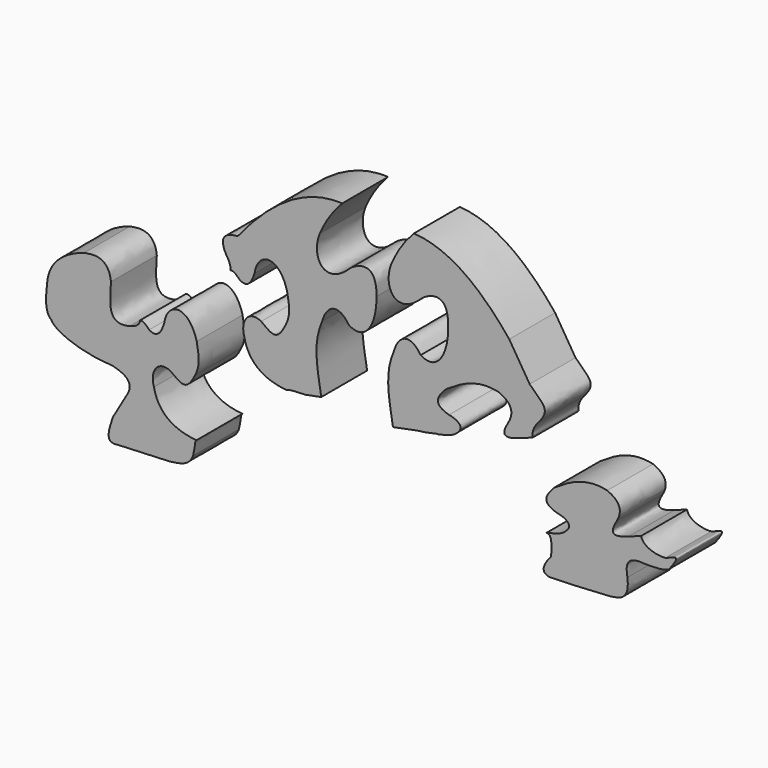
from build123d import *

# Parameters (mm, degrees)
F1_DEPTH = 12


with BuildPart() as f1:
    # F0 (on Front) → F1 (new body)
    with BuildSketch(Plane.XZ):
        with BuildLine():
            add(Edge.make_bspline(
                [(-45.8449507755, -30.2722072455), (-45.0373038776, -30.1761162576), (-44.6484686549, -30.7578016467), (-43.941360189, -31.4056891493)],
                knots=[0.0138164207, 0.0138164207, 0.0138164207, 0.0138164207, 0.9928004802, 0.9928004802, 0.9928004802, 0.9928004802], degree=3))
            add(Edge.make_bspline(
                [(-48.0757471404, -32.0822951013), (-46.6881017023, -31.7283579413), (-45.9495435845, -31.1383058377), (-45.8449507755, -30.2722072455)],
                knots=[0, 0, 0, 0, 0.5631001463, 0.5631001463, 0.5631001463, 0.5631001463], degree=3))
            add(Edge.make_bspline(
                [(-51.9596131404, -25.1498021013), (-52.0998001404, -29.0032331013), (-52.9532851404, -33.2183801013), (-48.0757471404, -32.0822951013)],
                knots=[0, 0, 0, 0, 1, 1, 1, 1], degree=3))
            add(Edge.make_bspline(
                [(-57.5557201404, -21.6417971013), (-56.1260271404, -21.4227111013), (-52.4818251404, -20.5015511013), (-51.9596131404, -25.1498021013)],
                knots=[0, 0, 0, 0, 1, 1, 1, 1], degree=3))
            add(Edge.make_bspline(
                [(-65.3234511404, -29.8271471013), (-65.0594941404, -25.9076961013), (-62.3853321404, -23.2227411013), (-57.5557201404, -21.6417971013)],
                knots=[0, 0, 0, 0, 1, 1, 1, 1], degree=3))
            add(Edge.make_bspline(
                [(-64.4464501404, -36.2167321013), (-65.7482111404, -35.2981831013), (-65.6745951404, -32.7291821013), (-65.3234511404, -29.8271471013)],
                knots=[0, 0, 0, 0, 1, 1, 1, 1], degree=3))
            add(Edge.make_bspline(
                [(-51.5002301404, -40.5599791013), (-58.8537851404, -40.1618431013), (-63.7433521404, -37.8487831013), (-64.4464501404, -36.2167321013)],
                knots=[0, 0, 0, 0, 1, 1, 1, 1], degree=3))
            add(Edge.make_bspline(
                [(-48.3680811404, -44.4856091013), (-46.9755981404, -41.7222641013), (-50.1851831404, -40.9703021013), (-51.5002301404, -40.5599791013)],
                knots=[0, 0, 0, 0, 1, 1, 1, 1], degree=3))
            Line((-48.3680811404, -44.4856091013), (-51.5419931404, -49.9564301013))
            add(Edge.make_bspline(
                [(-50.6649911404, -54.7590591013), (-53.3456761404, -55.1932241013), (-52.4255291404, -52.5592301013), (-51.5419931404, -49.9564301013)],
                knots=[0, 0, 0, 0, 1, 1, 1, 1], degree=3))
            Line((-50.6649911404, -54.7590591013), (-39.6369361507, -54.2805532244))
            add(Edge.make_bspline(
                [(-34.7507801507, -51.6077842244), (-35.6369361507, -54.0036222244), (-37.8110571507, -53.9730942244), (-39.6369361507, -54.2805532244)],
                knots=[0, 0, 0, 0, 1, 1, 1, 1], degree=3))
            add(Edge.make_bspline(
                [(-34.0284567295, -48.5307527398), (-34.4745798989, -48.8886475977), (-34.2730056498, -49.6825430518), (-34.7507801507, -51.6077842244)],
                knots=[0.4766943603, 0.4766943603, 0.4766943603, 0.4766943603, 0.9954393419, 0.9954393419, 0.9954393419, 0.9954393419], degree=3))
            add(Edge.make_bspline(
                [(-42.959955189, -41.6373791493), (-42.0418390729, -46.1886284081), (-38.5284702823, -48.1795127961), (-34.0284567295, -48.5307527398)],
                knots=[0, 0, 0, 0, 0.9845136883, 0.9845136883, 0.9845136883, 0.9845136883], degree=3))
            add(Edge.make_bspline(
                [(-39.431065189, -37.6073471493), (-42.009885189, -36.2487441493), (-43.877970189, -38.7036141493), (-42.959955189, -41.6373791493)],
                knots=[0, 0, 0, 0, 1, 1, 1, 1], degree=3))
            add(Edge.make_bspline(
                [(-34.294339189, -36.5632971493), (-36.196497189, -40.4302951493), (-37.241376189, -39.1889491493), (-39.431065189, -37.6073471493)],
                knots=[0, 0, 0, 0, 1, 1, 1, 1], degree=3))
            add(Edge.make_bspline(
                [(-34.002007189, -30.3198791493), (-33.615278189, -32.3526011493), (-33.151711189, -34.3776391493), (-34.294339189, -36.5632971493)],
                knots=[0, 0, 0, 0, 1, 1, 1, 1], degree=3))
            add(Edge.make_bspline(
                [(-40.809210189, -29.1505421493), (-40.138114189, -24.6796841493), (-35.639198189, -24.2694741493), (-34.002007189, -30.3198791493)],
                knots=[0, 0, 0, 0, 1, 1, 1, 1], degree=3))
            add(Edge.make_bspline(
                [(-43.941360189, -31.4056891493), (-42.081064189, -32.5779841493), (-41.316846189, -30.7279271493), (-40.809210189, -29.1505421493)],
                knots=[0, 0, 0, 0, 1, 1, 1, 1], degree=3))
        make_face()
    extrude(amount=F1_DEPTH)


with BuildPart() as f1b:
    # F0 (on Front) → F1, piece 2 (new body)
    with BuildSketch(Plane.XZ):
        with BuildLine():
            add(Edge.make_bspline(
                [(-3.5493105797, 5.0215643728), (-5.8036935797, 2.7199413728), (-7.1759255797, 0.3343053728), (-8.2684195797, -2.0779746272)],
                knots=[0, 0, 0, 0, 1, 1, 1, 1], degree=3))
            add(Edge.make_bspline(
                [(-25.4296236107, -8.1543007714), (-18.3372787343, 0.7478813145), (-11.0568971369, 5.4326630198), (-3.5493105797, 5.0215643728)],
                knots=[0, 0, 0, 0, 0.5368262438, 0.5368262438, 0.5368262438, 0.5368262438], degree=3))
            add(Edge.make_bspline(
                [(-27.8100566107, -12.3722607714), (-29.3184416107, -9.6427037714), (-28.3748066107, -8.3230577714), (-25.4296236107, -8.1543007714)],
                knots=[0, 0, 0, 0, 1, 1, 1, 1], degree=3))
            add(Edge.make_bspline(
                [(-26.9156442458, -14.9054209156), (-26.8344924591, -14.2334297064), (-27.134984297, -13.3952600313), (-27.8100566107, -12.3722607714)],
                knots=[0.5631001463, 0.5631001463, 0.5631001463, 0.5631001463, 1, 1, 1, 1], degree=3))
            add(Edge.make_bspline(
                [(-26.9156442458, -14.9054209156), (-26.1079973479, -14.8093299277), (-25.7191621253, -15.3910153168), (-25.0120536594, -16.0389028194)],
                knots=[0.0138164207, 0.0138164207, 0.0138164207, 0.0138164207, 0.9928004802, 0.9928004802, 0.9928004802, 0.9928004802], degree=3))
            add(Edge.make_bspline(
                [(-25.0120536594, -16.0389028194), (-23.1517576594, -17.2111978194), (-22.3875396594, -15.3611408194), (-21.8799036594, -13.7837558194)],
                knots=[0, 0, 0, 0, 1, 1, 1, 1], degree=3))
            add(Edge.make_bspline(
                [(-21.8799036594, -13.7837558194), (-21.2088076594, -9.3128978194), (-16.7098916594, -8.9026878194), (-15.0727006594, -14.9530928194)],
                knots=[0, 0, 0, 0, 1, 1, 1, 1], degree=3))
            add(Edge.make_bspline(
                [(-15.0727006594, -14.9530928194), (-14.6859716594, -16.9858148194), (-14.2224046594, -19.0108528194), (-15.3650326594, -21.1965108194)],
                knots=[0, 0, 0, 0, 1, 1, 1, 1], degree=3))
            add(Edge.make_bspline(
                [(-15.3650326594, -21.1965108194), (-17.2671906594, -25.0635088194), (-18.3120696594, -23.8221628194), (-20.5017586594, -22.2405608194)],
                knots=[0, 0, 0, 0, 1, 1, 1, 1], degree=3))
            add(Edge.make_bspline(
                [(-20.5017586594, -22.2405608194), (-23.0805786594, -20.8819578194), (-24.9486636594, -23.3368278194), (-24.0306486594, -26.2705928194)],
                knots=[0, 0, 0, 0, 1, 1, 1, 1], degree=3))
            add(Edge.make_bspline(
                [(-24.0306486594, -26.2705928194), (-23.1125325433, -30.8218420782), (-19.5991637527, -32.8127264662), (-15.0991501999, -33.1639664098)],
                knots=[0, 0, 0, 0, 0.9845136883, 0.9845136883, 0.9845136883, 0.9845136883], degree=3))
            add(Edge.make_bspline(
                [(-11.2265906851, -32.7437242637), (-13.7393281571, -32.8740949128), (-14.6907009874, -32.8362948542), (-15.0991501999, -33.1639664098)],
                knots=[0.0017560612, 0.0017560612, 0.0017560612, 0.0017560612, 0.4766943603, 0.4766943603, 0.4766943603, 0.4766943603], degree=3))
            Line((-11.2265906851, -32.7437242637), (-7.9269410512, -32.0941016145))
            add(Edge.make_bspline(
                [(-7.7255115797, -18.0310576272), (-9.8693992766, -22.8725708581), (-8.6456012061, -27.4646273112), (-7.9269410512, -32.0941016145)],
                knots=[0, 0, 0, 0, 0.9940362568, 0.9940362568, 0.9940362568, 0.9940362568], degree=3))
            add(Edge.make_bspline(
                [(-2.1294025797, -16.9452466272), (-4.3299685797, -13.6541016272), (-6.7549575797, -14.6530776272), (-7.7255115797, -18.0310576272)],
                knots=[0, 0, 0, 0, 1, 1, 1, 1], degree=3))
            add(Edge.make_bspline(
                [(3.6337524203, -9.8039436272), (3.7521504203, -14.4072226272), (1.6753304203, -19.2400576272), (-2.1294025797, -16.9452466272)],
                knots=[0, 0, 0, 0, 1, 1, 1, 1], degree=3))
            add(Edge.make_bspline(
                [(-1.8788315797, -6.3794626272), (-0.9089895797, -5.5503496272), (3.7205524203, -2.8571906272), (3.6337524203, -9.8039436272)],
                knots=[0, 0, 0, 0, 1, 1, 1, 1], degree=3))
            add(Edge.make_bspline(
                [(-8.2684195797, -2.0779746272), (-10.1702215797, -6.9599876272), (-7.1271355797, -11.5631846272), (-1.8788315797, -6.3794626272)],
                knots=[0, 0, 0, 0, 1, 1, 1, 1], degree=3))
        make_face()
    extrude(amount=F1_DEPTH)


with BuildPart() as f1c:
    # F0 (on Front) → F1, piece 3 (new body)
    with BuildSketch(Plane.XZ):
        with BuildLine():
            add(Edge.make_bspline(
                [(16.5388024374, -31.0114478382), (15.7269186174, -30.9559227169), (14.3985222109, -31.5607520701), (12.4413752168, -31.6893704477)],
                knots=[0.5229554083, 0.5229554083, 0.5229554083, 0.5229554083, 1, 1, 1, 1], degree=3))
            add(Edge.make_bspline(
                [(16.5388024374, -31.0114478382), (17.9833314374, -30.6849958382), (19.7451604374, -30.3481968382), (20.6419214374, -29.3096478382)],
                knots=[0, 0, 0, 0, 1, 1, 1, 1], degree=3))
            add(Edge.make_bspline(
                [(20.6419214374, -29.3096478382), (22.1740354374, -27.9142338382), (20.4187234374, -26.9375248382), (18.8043924374, -26.6786428382)],
                knots=[0, 0, 0, 0, 1, 1, 1, 1], degree=3))
            add(Edge.make_bspline(
                [(18.8043924374, -26.6786428382), (15.0581294374, -25.5653128382), (16.5932204374, -23.8591748382), (18.1779634374, -22.1474658382)],
                knots=[0, 0, 0, 0, 1, 1, 1, 1], degree=3))
            add(Edge.make_bspline(
                [(18.1779634374, -22.1474658382), (21.4855234374, -19.9038728382), (24.9269094374, -18.0989398382), (29.2240114374, -19.0988388382)],
                knots=[0, 0, 0, 0, 1, 1, 1, 1], degree=3))
            add(Edge.make_bspline(
                [(29.2240114374, -19.0988388382), (31.7774794374, -20.1628568382), (32.5377154374, -21.7726378382), (31.2494664374, -24.0058738382)],
                knots=[0, 0, 0, 0, 1, 1, 1, 1], degree=3))
            add(Edge.make_bspline(
                [(31.2494664374, -24.0058738382), (30.0865504374, -26.0272848382), (29.4806334374, -27.6792608382), (33.6925434374, -26.1357368382)],
                knots=[0, 0, 0, 0, 1, 1, 1, 1], degree=3))
            Line((33.6925434374, -26.1357368382), (36.3439928286, -25.154202191))
            add(Edge.make_bspline(
                [(36.3292402168, -24.8404014477), (36.3240759706, -24.9474945522), (36.3292336674, -25.0521376337), (36.3439928286, -25.154202191)],
                knots=[0, 0, 0, 0, 0.0596099248, 0.0596099248, 0.0596099248, 0.0596099248], degree=3))
            add(Edge.make_bspline(
                [(37.3732872168, -22.1258724477), (36.4599822168, -23.3034194477), (36.1830942168, -24.3473624477), (36.3292402168, -24.8404014477)],
                knots=[0, 0, 0, 0, 1, 1, 1, 1], degree=3))
            add(Edge.make_bspline(
                [(35.7028082168, -15.5274774477), (38.1129892168, -18.1712254477), (40.5076532168, -18.7420504477), (37.3732872168, -22.1258724477)],
                knots=[0, 0, 0, 0, 1, 1, 1, 1], degree=3))
            Line((35.7028082168, -15.5274774477), (31.4287997302, -8.6368724207))
            add(Edge.make_bspline(
                [(11.4635917612, 4.3719417235), (17.9411384634, 4.017245755), (24.5878220076, -0.1309462291), (31.4287997302, -8.6368724207)],
                knots=[0.5368262438, 0.5368262438, 0.5368262438, 0.5368262438, 1, 1, 1, 1], degree=3))
            add(Edge.make_bspline(
                [(11.4635917612, 4.3719417235), (9.2092087612, 2.0703187235), (7.8369767612, -0.3153172765), (6.7444827612, -2.7275972765)],
                knots=[0, 0, 0, 0, 1, 1, 1, 1], degree=3))
            add(Edge.make_bspline(
                [(6.7444827612, -2.7275972765), (4.8426807612, -7.6096102765), (7.8857667612, -12.2128072765), (13.1340707612, -7.0290852765)],
                knots=[0, 0, 0, 0, 1, 1, 1, 1], degree=3))
            add(Edge.make_bspline(
                [(13.1340707612, -7.0290852765), (14.1039127612, -6.1999722765), (18.7334547612, -3.5068132765), (18.6466547612, -10.4535662765)],
                knots=[0, 0, 0, 0, 1, 1, 1, 1], degree=3))
            add(Edge.make_bspline(
                [(18.6466547612, -10.4535662765), (18.7650527612, -15.0568452765), (16.6882327612, -19.8896802765), (12.8834997612, -17.5948692765)],
                knots=[0, 0, 0, 0, 1, 1, 1, 1], degree=3))
            add(Edge.make_bspline(
                [(12.8834997612, -17.5948692765), (10.6829337612, -14.3037242765), (8.2579447612, -15.3027002765), (7.2873907612, -18.6806802765)],
                knots=[0, 0, 0, 0, 1, 1, 1, 1], degree=3))
            add(Edge.make_bspline(
                [(7.2873907612, -18.6806802765), (5.1435030644, -23.5221935073), (6.3673011348, -28.1142499605), (7.0859612897, -32.7437242637)],
                knots=[0, 0, 0, 0, 0.9940362568, 0.9940362568, 0.9940362568, 0.9940362568], degree=3))
            Line((7.0859612897, -32.7437242637), (12.4413752168, -31.6893704477))
        make_face()
    extrude(amount=F1_DEPTH)


with BuildPart() as f1d:
    # F0 (on Front) → F1, piece 4 (new body)
    with BuildSketch(Plane.XZ):
        with BuildLine():
            add(Edge.make_bspline(
                [(39.2516157529, -41.757464416), (40.6961447529, -41.431012416), (42.4579737529, -41.094213416), (43.3547347529, -40.055664416)],
                knots=[0, 0, 0, 0, 1, 1, 1, 1], degree=3))
            add(Edge.make_bspline(
                [(40.2073915323, -45.8181080254), (40.410939897, -42.6727780793), (40.1416353485, -41.8183332803), (39.2516157529, -41.757464416)],
                knots=[0, 0, 0, 0, 0.5229554083, 0.5229554083, 0.5229554083, 0.5229554083], degree=3))
            add(Edge.make_bspline(
                [(39.8732945323, -49.7437380254), (37.5745945323, -49.2946740254), (38.9268615323, -47.3197620254), (40.2073915323, -45.8181080254)],
                knots=[0, 0, 0, 0, 1, 1, 1, 1], degree=3))
            add(Edge.make_bspline(
                [(52.4018945323, -49.1590690254), (45.7012145323, -49.6793940254), (42.7617685323, -49.5700100254), (39.8732945323, -49.7437380254)],
                knots=[0, 0, 0, 0, 1, 1, 1, 1], degree=3))
            add(Edge.make_bspline(
                [(56.1604745323, -44.4817240254), (56.7219125323, -48.6534310254), (54.5569355323, -48.8990950254), (52.4018945323, -49.1590690254)],
                knots=[0, 0, 0, 0, 1, 1, 1, 1], degree=3))
            add(Edge.make_bspline(
                [(59.8355295323, -40.8066690254), (55.6943895323, -40.3958150254), (55.8261315323, -42.3819430254), (56.1604745323, -44.4817240254)],
                knots=[0, 0, 0, 0, 1, 1, 1, 1], degree=3))
            add(Edge.make_bspline(
                [(64.9304925323, -40.0967160254), (64.1311635323, -40.8169080254), (61.5569745323, -40.8037140254), (59.8355295323, -40.8066690254)],
                knots=[0, 0, 0, 0, 1, 1, 1, 1], degree=3))
            add(Edge.make_bspline(
                [(64.0952535323, -38.3009500254), (65.1097015323, -38.1455500254), (68.1064355323, -35.9595190254), (64.9304925323, -40.0967160254)],
                knots=[0, 0, 0, 0, 1, 1, 1, 1], degree=3))
            add(Edge.make_bspline(
                [(59.0568061441, -35.9002187687), (59.2896426852, -37.5103616605), (61.9120307682, -38.4787777887), (64.0952535323, -38.3009500254)],
                knots=[0.0596099248, 0.0596099248, 0.0596099248, 0.0596099248, 1, 1, 1, 1], degree=3))
            Line((59.0568061441, -35.9002187687), (56.4053567529, -36.881753416))
            add(Edge.make_bspline(
                [(53.9622797529, -34.751890416), (52.7993637529, -36.773301416), (52.1934467529, -38.425277416), (56.4053567529, -36.881753416)],
                knots=[0, 0, 0, 0, 1, 1, 1, 1], degree=3))
            add(Edge.make_bspline(
                [(51.9368247529, -29.844855416), (54.4902927529, -30.908873416), (55.2505287529, -32.518654416), (53.9622797529, -34.751890416)],
                knots=[0, 0, 0, 0, 1, 1, 1, 1], degree=3))
            add(Edge.make_bspline(
                [(40.8907767529, -32.893482416), (44.1983367529, -30.649889416), (47.6397227529, -28.844956416), (51.9368247529, -29.844855416)],
                knots=[0, 0, 0, 0, 1, 1, 1, 1], degree=3))
            add(Edge.make_bspline(
                [(41.5172057529, -37.424659416), (37.7709427529, -36.311329416), (39.3060337529, -34.605191416), (40.8907767529, -32.893482416)],
                knots=[0, 0, 0, 0, 1, 1, 1, 1], degree=3))
            add(Edge.make_bspline(
                [(43.3547347529, -40.055664416), (44.8868487529, -38.660250416), (43.1315367529, -37.683541416), (41.5172057529, -37.424659416)],
                knots=[0, 0, 0, 0, 1, 1, 1, 1], degree=3))
        make_face()
    extrude(amount=F1_DEPTH)


solid = Compound([f1.part, f1b.part, f1c.part, f1d.part])
